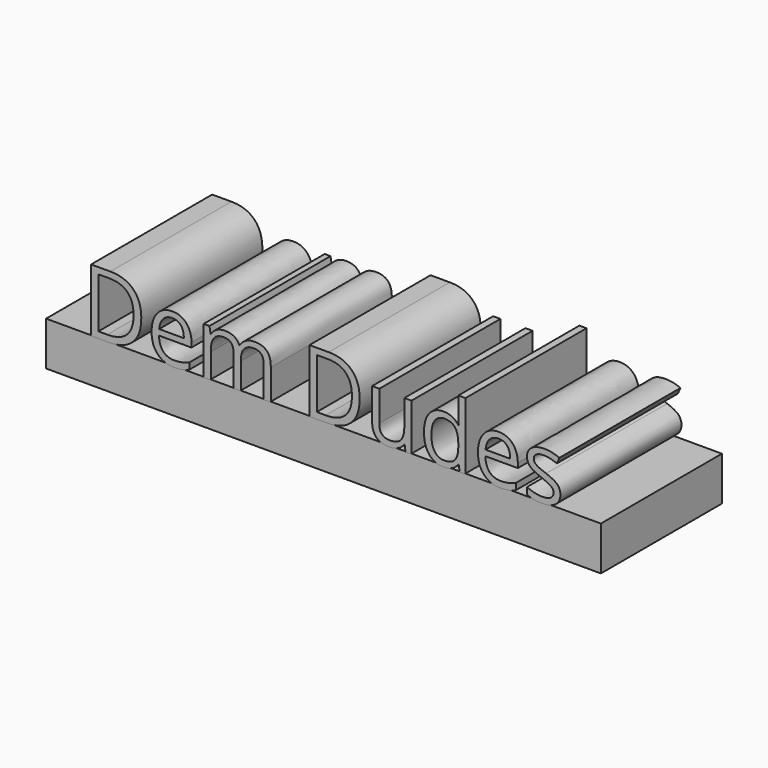
from build123d import *

# Parameters (mm, degrees)
F1_DEPTH     = 25.4
F4_TEXT_SIZE = 14.7801746304
F5_DEPTH     = 25.4


# Not quite as in the source:
# - the program builds the solid bodies; features that only make, move or delete a surface that nothing else refers to are left out
# - Text() gives the source's letters only with a copy of the font that has no kerning and outlines rounded to 1/6400 em; it was checked with that copy


with BuildPart() as f1:
    # F0 (on Front) → F1 (new body)
    with BuildSketch(Plane.XZ):
        Polygon((-56.1646558344, 27.4758059531), (-56.1646558344, 20.1010350138), (36.967549473, 20.1010350138), (36.967549473, 27.4758059531), (-41.7786203325, 27.4758059531), (-55.5734522641, 27.4758059531), align=None)
    extrude(amount=F1_DEPTH)


with BuildPart() as f5:
    # F4 (on Front) → F5 (new body)
    with BuildSketch(Plane.XZ):
        with Locations((-50.0555187464, 27.3925866932)):
            Text('Dem Dudes', F4_TEXT_SIZE, font='Open Sans', text_align=(TextAlign.LEFT, TextAlign.BOTTOM))
    extrude(amount=F5_DEPTH)


solid = Compound([f1.part, f5.part])
